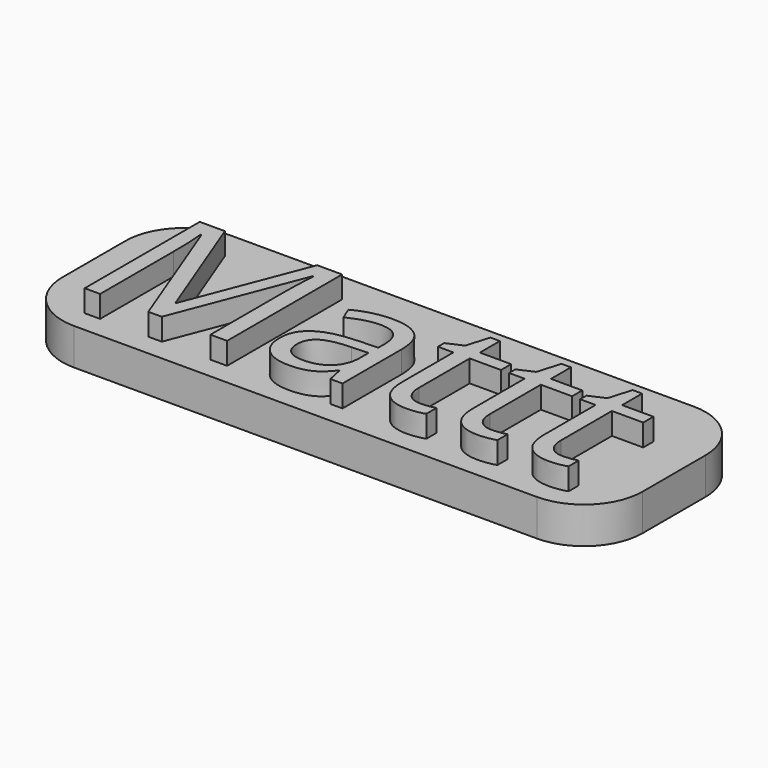
from build123d import *

# Parameters (mm, degrees)
F0_W         = 79.2141482234
F0_H         = 26.7467630528
F0_TEXT_SIZE = 27.5049125776
F1_DEPTH     = 5
F2_DEPTH     = 8
F3_R         = 8


# Not quite as in the source:
# - Text() gives the source's letters only with a copy of the font that has no kerning and outlines rounded to 1/6400 em; it was checked with that copy


with BuildPart() as f1:
    # F0 (on Top) → F1 (new body)
    with BuildSketch(Plane.XY):
        Rectangle(F0_W, F0_H)
        with BuildLine():
            Line((-22.0469056148, -10.3659136221), (-23.8862966435, -10.3659136221))
            Line((-23.8862966435, -10.3659136221), (-30.5476426583, 7.0395388684))
            Line((-30.5476426583, 7.0395388684), (-30.6550837231, 7.0395388684))
            add(Edge.make_bspline(
                [(-30.6550837231, 7.0395388684), (-30.4659874491, 4.9723727825), (-30.4659874491, 2.1230357452)],
                knots=[0, 0, 0, 1, 1, 1], degree=2))
            Line((-30.4659874491, 2.1230357452), (-30.4659874491, -10.3659136221))
            Line((-30.4659874491, -10.3659136221), (-32.5761299609, -10.3659136221))
            Line((-32.5761299609, -10.3659136221), (-32.5761299609, 9.2700153727))
            Line((-32.5761299609, 9.2700153727), (-29.1380158887, 9.2700153727))
            Line((-29.1380158887, 9.2700153727), (-22.9193270607, -6.9277995499))
            Line((-22.9193270607, -6.9277995499), (-22.8118859959, -6.9277995499))
            Line((-22.8118859959, -6.9277995499), (-16.5416254567, 9.2700153727))
            Line((-16.5416254567, 9.2700153727), (-13.1292972401, 9.2700153727))
            Line((-13.1292972401, 9.2700153727), (-13.1292972401, -10.3659136221))
            Line((-13.1292972401, -10.3659136221), (-15.4113454555, -10.3659136221))
            Line((-15.4113454555, -10.3659136221), (-15.4113454555, 2.2863461636))
            add(Edge.make_bspline(
                [(-15.4113454555, 2.2863461636), (-15.4113454555, 4.4609533143), (-15.2222491815, 7.0137530129)],
                knots=[0, 0, 0, 1, 1, 1], degree=2))
            Line((-15.2222491815, 7.0137530129), (-15.3296902463, 7.0137530129))
            Line((-15.3296902463, 7.0137530129), (-22.0469056148, -10.3659136221))
        make_face(mode=Mode.SUBTRACT)
        with BuildLine():
            Line((2.6258604958, -10.3659136221), (0.9712680985, -10.3659136221))
            Line((0.9712680985, -10.3659136221), (0.5286109117, -8.268664038))
            Line((0.5286109117, -8.268664038), (0.421169847, -8.268664038))
            add(Edge.make_bspline(
                [(0.421169847, -8.268664038), (-0.6790266561, -9.6525049521), (-1.7727766954, -10.1445850287)],
                knots=[0, 0, 0, 1, 1, 1], degree=2))
            add(Edge.make_bspline(
                [(-1.7727766954, -10.1445850287), (-2.8665267346, -10.6366651053), (-4.5082262041, -10.6366651053)],
                knots=[0, 0, 0, 1, 1, 1], degree=2))
            add(Edge.make_bspline(
                [(-4.5082262041, -10.6366651053), (-6.6957262825, -10.6366651053), (-7.9377449911, -9.506385104)],
                knots=[0, 0, 0, 1, 1, 1], degree=2))
            add(Edge.make_bspline(
                [(-7.9377449911, -9.506385104), (-9.1797636996, -8.3761051028), (-9.1797636996, -6.2960460891)],
                knots=[0, 0, 0, 1, 1, 1], degree=2))
            add(Edge.make_bspline(
                [(-9.1797636996, -6.2960460891), (-9.1797636996, -1.839390723), (-2.0499746424, -1.6245085935)],
                knots=[0, 0, 0, 1, 1, 1], degree=2))
            Line((-2.0499746424, -1.6245085935), (0.4469557025, -1.5428533843))
            Line((0.4469557025, -1.5428533843), (0.4469557025, -0.6274555126))
            add(Edge.make_bspline(
                [(0.4469557025, -0.6274555126), (0.4469557025, 1.1044944513), (-0.2965364656, 1.9296418286)],
                knots=[0, 0, 0, 1, 1, 1], degree=2))
            add(Edge.make_bspline(
                [(-0.2965364656, 1.9296418286), (-1.0400286337, 2.7547892059), (-2.6817281032, 2.7547892059)],
                knots=[0, 0, 0, 1, 1, 1], degree=2))
            add(Edge.make_bspline(
                [(-2.6817281032, 2.7547892059), (-4.5211191318, 2.7547892059), (-6.8418461306, 1.6288068473)],
                knots=[0, 0, 0, 1, 1, 1], degree=2))
            Line((-6.8418461306, 1.6288068473), (-7.529468945, 3.3349709556))
            add(Edge.make_bspline(
                [(-7.529468945, 3.3349709556), (-6.4421653697, 3.9237479905), (-5.1464261287, 4.2589641125)],
                knots=[0, 0, 0, 1, 1, 1], degree=2))
            add(Edge.make_bspline(
                [(-5.1464261287, 4.2589641125), (-3.8506868877, 4.5941802346), (-2.5442035403, 4.5941802346)],
                knots=[0, 0, 0, 1, 1, 1], degree=2))
            add(Edge.make_bspline(
                [(-2.5442035403, 4.5941802346), (0.0859537249, 4.5941802346), (1.3559071103, 3.4273702713)],
                knots=[0, 0, 0, 1, 1, 1], degree=2))
            add(Edge.make_bspline(
                [(1.3559071103, 3.4273702713), (2.6258604958, 2.2605603081), (2.6258604958, -0.3180252461)],
                knots=[0, 0, 0, 1, 1, 1], degree=2))
            Line((2.6258604958, -0.3180252461), (2.6258604958, -10.3659136221))
        make_face(mode=Mode.SUBTRACT)
        with BuildLine():
            add(Edge.make_bspline(
                [(10.2369855231, -8.0817165854), (10.8687389838, -8.7929764341), (11.9689354869, -8.7929764341)],
                knots=[0, 0, 0, 1, 1, 1], degree=2))
            add(Edge.make_bspline(
                [(11.9689354869, -8.7929764341), (12.5620101644, -8.7929764341), (13.112108416, -8.7070235822)],
                knots=[0, 0, 0, 1, 1, 1], degree=2))
            add(Edge.make_bspline(
                [(13.112108416, -8.7070235822), (13.6622066675, -8.6210707304), (13.9845298618, -8.5265225935)],
                knots=[0, 0, 0, 1, 1, 1], degree=2))
            Line((13.9845298618, -8.5265225935), (13.9845298618, -10.2326867018))
            add(Edge.make_bspline(
                [(13.9845298618, -10.2326867018), (13.6235278842, -10.4045924054), (12.9187144994, -10.5206287553)],
                knots=[0, 0, 0, 1, 1, 1], degree=2))
            add(Edge.make_bspline(
                [(12.9187144994, -10.5206287553), (12.2139011146, -10.6366651053), (11.6466122927, -10.6366651053)],
                knots=[0, 0, 0, 1, 1, 1], degree=2))
            add(Edge.make_bspline(
                [(11.6466122927, -10.6366651053), (7.3790532006, -10.6366651053), (7.3790532006, -6.1370333133)],
                knots=[0, 0, 0, 1, 1, 1], degree=2))
            Line((7.3790532006, -6.1370333133), (7.3790532006, 2.6215622856))
            Line((7.3790532006, 2.6215622856), (5.2689106888, 2.6215622856))
            Line((5.2689106888, 2.6215622856), (5.2689106888, 3.6959729332))
            Line((5.2689106888, 3.6959729332), (7.3790532006, 4.6242637327))
            Line((7.3790532006, 4.6242637327), (8.3159392852, 7.7658404662))
            Line((8.3159392852, 7.7658404662), (9.6052320623, 7.7658404662))
            Line((9.6052320623, 7.7658404662), (9.6052320623, 4.3535122495))
            Line((9.6052320623, 4.3535122495), (13.877088797, 4.3535122495))
            Line((13.877088797, 4.3535122495), (13.877088797, 2.6215622856))
            Line((13.877088797, 2.6215622856), (9.6052320623, 2.6215622856))
            Line((9.6052320623, 2.6215622856), (9.6052320623, -6.0424851763))
            add(Edge.make_bspline(
                [(9.6052320623, -6.0424851763), (9.6052320623, -7.3704567367), (10.2369855231, -8.0817165854)],
                knots=[0, 0, 0, 1, 1, 1], degree=2))
        make_face(mode=Mode.SUBTRACT)
        with BuildLine():
            add(Edge.make_bspline(
                [(19.9453601344, -8.0817165854), (20.5771135952, -8.7929764341), (21.6773100983, -8.7929764341)],
                knots=[0, 0, 0, 1, 1, 1], degree=2))
            add(Edge.make_bspline(
                [(21.6773100983, -8.7929764341), (22.2703847758, -8.7929764341), (22.8204830273, -8.7070235822)],
                knots=[0, 0, 0, 1, 1, 1], degree=2))
            add(Edge.make_bspline(
                [(22.8204830273, -8.7070235822), (23.3705812789, -8.6210707304), (23.6929044731, -8.5265225935)],
                knots=[0, 0, 0, 1, 1, 1], degree=2))
            Line((23.6929044731, -8.5265225935), (23.6929044731, -10.2326867018))
            add(Edge.make_bspline(
                [(23.6929044731, -10.2326867018), (23.3319024956, -10.4045924054), (22.6270891108, -10.5206287553)],
                knots=[0, 0, 0, 1, 1, 1], degree=2))
            add(Edge.make_bspline(
                [(22.6270891108, -10.5206287553), (21.922275726, -10.6366651053), (21.354986904, -10.6366651053)],
                knots=[0, 0, 0, 1, 1, 1], degree=2))
            add(Edge.make_bspline(
                [(21.354986904, -10.6366651053), (17.0874278119, -10.6366651053), (17.0874278119, -6.1370333133)],
                knots=[0, 0, 0, 1, 1, 1], degree=2))
            Line((17.0874278119, -6.1370333133), (17.0874278119, 2.6215622856))
            Line((17.0874278119, 2.6215622856), (14.9772853001, 2.6215622856))
            Line((14.9772853001, 2.6215622856), (14.9772853001, 3.6959729332))
            Line((14.9772853001, 3.6959729332), (17.0874278119, 4.6242637327))
            Line((17.0874278119, 4.6242637327), (18.0243138966, 7.7658404662))
            Line((18.0243138966, 7.7658404662), (19.3136066737, 7.7658404662))
            Line((19.3136066737, 7.7658404662), (19.3136066737, 4.3535122495))
            Line((19.3136066737, 4.3535122495), (23.5854634084, 4.3535122495))
            Line((23.5854634084, 4.3535122495), (23.5854634084, 2.6215622856))
            Line((23.5854634084, 2.6215622856), (19.3136066737, 2.6215622856))
            Line((19.3136066737, 2.6215622856), (19.3136066737, -6.0424851763))
            add(Edge.make_bspline(
                [(19.3136066737, -6.0424851763), (19.3136066737, -7.3704567367), (19.9453601344, -8.0817165854)],
                knots=[0, 0, 0, 1, 1, 1], degree=2))
        make_face(mode=Mode.SUBTRACT)
        with BuildLine():
            add(Edge.make_bspline(
                [(29.6537347458, -8.0817165854), (30.2854882066, -8.7929764341), (31.3856847097, -8.7929764341)],
                knots=[0, 0, 0, 1, 1, 1], degree=2))
            add(Edge.make_bspline(
                [(31.3856847097, -8.7929764341), (31.9787593871, -8.7929764341), (32.5288576387, -8.7070235822)],
                knots=[0, 0, 0, 1, 1, 1], degree=2))
            add(Edge.make_bspline(
                [(32.5288576387, -8.7070235822), (33.0789558902, -8.6210707304), (33.4012790845, -8.5265225935)],
                knots=[0, 0, 0, 1, 1, 1], degree=2))
            Line((33.4012790845, -8.5265225935), (33.4012790845, -10.2326867018))
            add(Edge.make_bspline(
                [(33.4012790845, -10.2326867018), (33.0402771069, -10.4045924054), (32.3354637221, -10.5206287553)],
                knots=[0, 0, 0, 1, 1, 1], degree=2))
            add(Edge.make_bspline(
                [(32.3354637221, -10.5206287553), (31.6306503373, -10.6366651053), (31.0633615154, -10.6366651053)],
                knots=[0, 0, 0, 1, 1, 1], degree=2))
            add(Edge.make_bspline(
                [(31.0633615154, -10.6366651053), (26.7958024233, -10.6366651053), (26.7958024233, -6.1370333133)],
                knots=[0, 0, 0, 1, 1, 1], degree=2))
            Line((26.7958024233, -6.1370333133), (26.7958024233, 2.6215622856))
            Line((26.7958024233, 2.6215622856), (24.6856599115, 2.6215622856))
            Line((24.6856599115, 2.6215622856), (24.6856599115, 3.6959729332))
            Line((24.6856599115, 3.6959729332), (26.7958024233, 4.6242637327))
            Line((26.7958024233, 4.6242637327), (27.732688508, 7.7658404662))
            Line((27.732688508, 7.7658404662), (29.021981285, 7.7658404662))
            Line((29.021981285, 7.7658404662), (29.021981285, 4.3535122495))
            Line((29.021981285, 4.3535122495), (33.2938380197, 4.3535122495))
            Line((33.2938380197, 4.3535122495), (33.2938380197, 2.6215622856))
            Line((33.2938380197, 2.6215622856), (29.021981285, 2.6215622856))
            Line((29.021981285, 2.6215622856), (29.021981285, -6.0424851763))
            add(Edge.make_bspline(
                [(29.021981285, -6.0424851763), (29.021981285, -7.3704567367), (29.6537347458, -8.0817165854)],
                knots=[0, 0, 0, 1, 1, 1], degree=2))
        make_face(mode=Mode.SUBTRACT)
        with Locations((-35.2750495076, -10.3659136221)):
            Text('Mattt', F0_TEXT_SIZE, font='Open Sans', text_align=(TextAlign.LEFT, TextAlign.BOTTOM))
        with BuildLine():
            add(Edge.make_bspline(
                [(-6.1112468902, -8.1633717946), (-5.3806476499, -8.7929764341), (-4.0655690173, -8.7929764341)],
                knots=[0, 0, 0, 1, 1, 1], degree=2))
            add(Edge.make_bspline(
                [(-4.0655690173, -8.7929764341), (-1.981212361, -8.7929764341), (-0.7929141848, -7.6519523263)],
                knots=[0, 0, 0, 1, 1, 1], degree=2))
            add(Edge.make_bspline(
                [(-0.7929141848, -7.6519523263), (0.3953839914, -6.5109282186), (0.3953839914, -4.4566550605)],
                knots=[0, 0, 0, 1, 1, 1], degree=2))
            Line((0.3953839914, -4.4566550605), (0.3953839914, -3.1286835001))
            Line((0.3953839914, -3.1286835001), (-1.8350925129, -3.2189339945))
            add(Edge.make_bspline(
                [(-1.8350925129, -3.2189339945), (-4.4953332763, -3.3134821315), (-5.6685897034, -4.0462301931)],
                knots=[0, 0, 0, 1, 1, 1], degree=2))
            add(Edge.make_bspline(
                [(-5.6685897034, -4.0462301931), (-6.8418461306, -4.7789782548), (-6.8418461306, -6.3218319447)],
                knots=[0, 0, 0, 1, 1, 1], degree=2))
            add(Edge.make_bspline(
                [(-6.8418461306, -6.3218319447), (-6.8418461306, -7.5337671551), (-6.1112468902, -8.1633717946)],
                knots=[0, 0, 0, 1, 1, 1], degree=2))
        make_face()
    extrude(amount=F1_DEPTH)

    # F0 (on Top) → F2 (join)
    with BuildSketch(Plane.XY):
        with Locations((-35.2750495076, -10.3659136221)):
            Text('Mattt', F0_TEXT_SIZE, font='Open Sans', text_align=(TextAlign.LEFT, TextAlign.BOTTOM))
    extrude(amount=F2_DEPTH)

    # F3
    f3_edges = [f1.edges().sort_by_distance(p)[0] for p in [
        (-39.607074, -13.373382, 2.5),
        (-39.607074, 13.373382, 2.5),
        (39.607074, -13.373382, 2.5),
        (39.607074, 13.373382, 2.5),
    ]]
    fillet(f3_edges, radius=F3_R)


solid = f1.part
